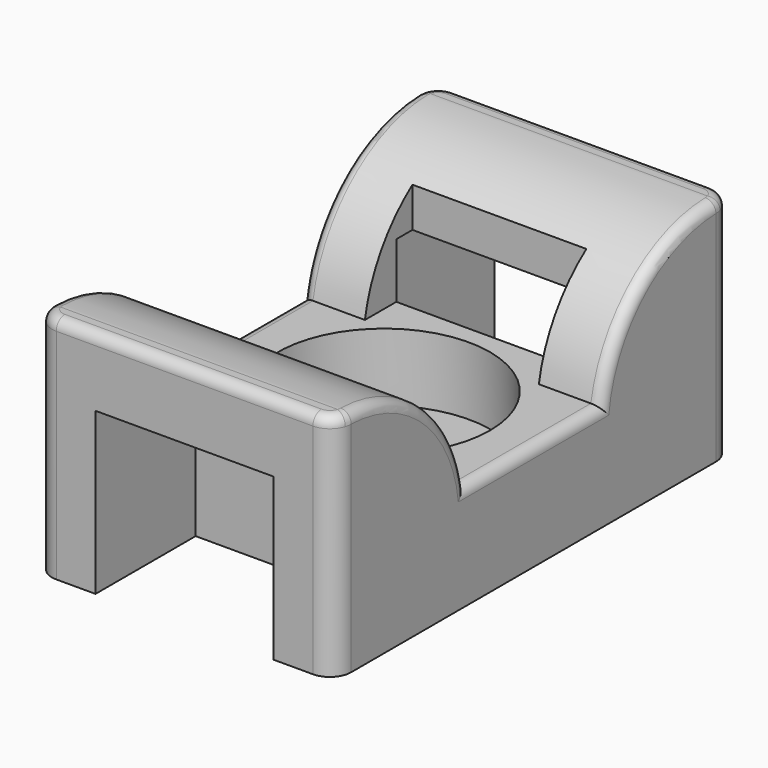
from build123d import *

# Parameters (mm, degrees)
F0_W         = 14.1
F0_H         = 23.5
F1_DEPTH     = 10.8
F2_W         = 8.2
F2_H         = 2.8
F2_H_2       = 8
F2_W_2       = 2.95
F3_DEPTH     = 5.8
F4_W         = 8.4
F4_H         = 5.9
F5_DEPTH     = 7.6
F6_R         = 5
F7_DEPTH     = 3.2
F8_R         = 2.7
F9_DEPTH     = 1.801
F10_T1_DEPTH = 37.4318792991
F11_R        = 1
F12_R        = 0.5


# Not quite as in the source:
# - a fillet or chamfer that OpenCascade refuses, or shapes differently, is made with other operations: its cross-section is extruded or revolved along the edge and cut away or added


with BuildPart() as f1:
    # F0 (on Top) → F1 (new body)
    with BuildSketch(Plane.XY):
        Rectangle(F0_W, F0_H)
    extrude(amount=F1_DEPTH)

    # F2 (on face) → F3 (cut)
    with BuildSketch(Plane.XY.offset(10.8)):
        with Locations((0, -5.4)):
            Rectangle(F2_W, F2_H)
        Rectangle(F2_W, F2_H_2)
        with Locations((5.575, 0)):
            Rectangle(F2_W_2, F2_H_2)
        with Locations((-5.575, 0)):
            Rectangle(F2_W_2, F2_H_2)
        with Locations((0, 5.4)):
            Rectangle(F2_W, F2_H)
    extrude(amount=-F3_DEPTH, mode=Mode.SUBTRACT)

    # F4 (on face) → F5 (cut)
    with BuildSketch(Plane(origin=(0, 0, 0), x_dir=(1, 0, 0), z_dir=(0, 0, -1))):
        with Locations((0, -8.8)):
            Rectangle(F4_W, F4_H)
        with Locations((0, 8.8)):
            Rectangle(F4_W, F4_H)
    extrude(amount=-F5_DEPTH, mode=Mode.SUBTRACT)

    # F6 (on face) → F7 (cut)
    with BuildSketch(Plane.XY.offset(5)):
        Circle(F6_R)
    extrude(amount=-F7_DEPTH, mode=Mode.SUBTRACT)

    # F8 (on face) → F9 (cut, through all)
    with BuildSketch(Plane.XY.offset(1.8)):
        Circle(F8_R)
    extrude(amount=-F9_DEPTH, mode=Mode.SUBTRACT)

    # F10: fillet of radius 7 on 2 edges, made by hand

    # F10_s2 → F10_t1 (cut)
    with BuildSketch(Plane.YZ.offset(-24.2909396496)):
        with BuildLine():
            ThreePointArc((-10.8963758598, 10.8), (-6.3908237294, 9.1572380944), (-4, 5))
            Line((-4, 5), (-4, 10.8))
            Line((-4, 10.8), (-10.8963758598, 10.8))
        make_face()
        with BuildLine():
            ThreePointArc((10.8963758598, 10.8), (6.3908237294, 9.1572380944), (4, 5))
            Line((4, 5), (4, 10.8))
            Line((4, 10.8), (10.8963758598, 10.8))
        make_face()
    extrude(amount=F10_T1_DEPTH, mode=Mode.SUBTRACT)

    # F11
    f11_edges = [f1.edges().sort_by_distance(p)[0] for p in [
        (7.05, -11.75, 5.4),
        (-7.05, -11.75, 5.4),
        (7.05, 11.75, 5.4),
        (-7.05, 11.75, 5.4),
    ]]
    fillet(f11_edges, radius=F11_R)

    # F12
    f12_edges = [f1.edges().sort_by_distance(p)[0] for p in [
        (0, 11.75, 10.8),
        (0, -11.75, 10.8),
        (-7.05, 0, 5),
        (7.05, 0, 5),
        (7.05, -6.335055, 9.109835),
        (7.05, 6.335055, 9.109835),
        (7.047304, -10.823382, 10.79962),
        (6.703309, -11.507092, 10.8),
        (7.047304, 10.823382, 10.79962),
        (6.703309, 11.507092, 10.8),
        (-7.05, -6.335055, 9.109835),
        (-7.047304, -10.823382, 10.799619),
        (-7.05, 6.335055, 9.109835),
        (-7.047304, 10.823382, 10.79962),
        (-6.703309, -11.507092, 10.8),
        (-6.703309, 11.507092, 10.8),
    ]]
    fillet(f12_edges, radius=F12_R)


solid = f1.part
